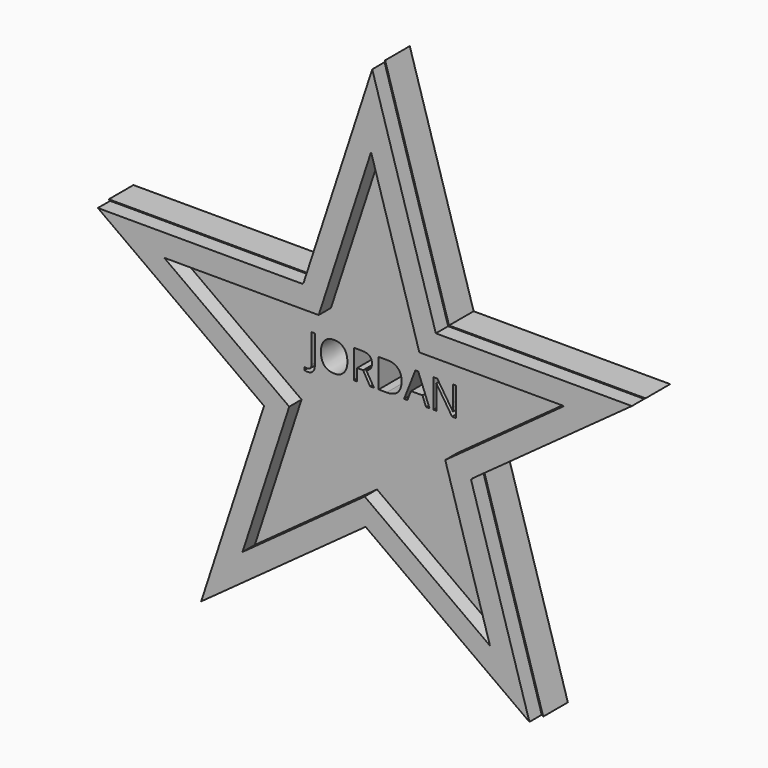
from build123d import *

# Parameters (mm, degrees)
F1_DEPTH = 6.35
F3_DEPTH = 3.175


with BuildPart() as f1:
    # F0 (on Front) → F1 (new body)
    with BuildSketch(Plane.XZ):
        Polygon((36.4045640823, 1.9488933967), (69.6907226001, 26.065217087), (29.1461811696, 26.1190709712), (15.9708538221, 69.9924798862), (1.6629783111, 26.15557594), (-41.0424164863, 26.2123000095), (-6.4774139305, 1.2147947246), (-19.4446871391, -38.5147311336), (14.4759376997, -13.9387270281), (48.5830571498, -38.6050899867), align=None)
        with BuildLine():
            add(Edge.make_bspline(
                [(1.0703261445, 8.6234759039), (0.6811166374, 8.1998862237), (-0.0492998709, 8.1998862237)],
                knots=[0, 0, 0, 1, 1, 1], degree=2))
            add(Edge.make_bspline(
                [(-0.0492998709, 8.1998862237), (-0.4294278228, 8.1998862237), (-0.6486825118, 8.3088648857)],
                knots=[0, 0, 0, 1, 1, 1], degree=2))
            Line((-0.6486825118, 8.3088648857), (-0.6486825118, 8.8965712414))
            add(Edge.make_bspline(
                [(-0.6486825118, 8.8965712414), (-0.3606674766, 8.81613461), (-0.0492998709, 8.81613461)],
                knots=[0, 0, 0, 1, 1, 1], degree=2))
            add(Edge.make_bspline(
                [(-0.0492998709, 8.81613461), (0.3528832864, 8.81613461), (0.5617590552, 9.0593905519)],
                knots=[0, 0, 0, 1, 1, 1], degree=2))
            add(Edge.make_bspline(
                [(0.5617590552, 9.0593905519), (0.7706348241, 9.3026464938), (0.7706348241, 9.7606163472)],
                knots=[0, 0, 0, 1, 1, 1], degree=2))
            Line((0.7706348241, 9.7606163472), (0.7706348241, 15.6882771403))
            Line((0.7706348241, 15.6882771403), (1.4595356516, 15.6882771403))
            Line((1.4595356516, 15.6882771403), (1.4595356516, 9.8177004082))
            add(Edge.make_bspline(
                [(1.4595356516, 9.8177004082), (1.4595356516, 9.0470655842), (1.0703261445, 8.6234759039)],
                knots=[0, 0, 0, 1, 1, 1], degree=2))
        make_face(mode=Mode.SUBTRACT)
        with BuildLine():
            add(Edge.make_bspline(
                [(7.4598488861, 14.9708342823), (8.1772917442, 14.1599811425), (8.1772917442, 12.7328796164)],
                knots=[0, 0, 0, 1, 1, 1], degree=2))
            add(Edge.make_bspline(
                [(8.1772917442, 12.7328796164), (8.1772917442, 11.3096701855), (7.4572541561, 10.4942762681)],
                knots=[0, 0, 0, 1, 1, 1], degree=2))
            add(Edge.make_bspline(
                [(7.4572541561, 10.4942762681), (6.7372165679, 9.6788823507), (5.4567172896, 9.6788823507)],
                knots=[0, 0, 0, 1, 1, 1], degree=2))
            add(Edge.make_bspline(
                [(5.4567172896, 9.6788823507), (4.1476759807, 9.6788823507), (3.4360712652, 10.4800052528)],
                knots=[0, 0, 0, 1, 1, 1], degree=2))
            add(Edge.make_bspline(
                [(3.4360712652, 10.4800052528), (2.7244665497, 11.2811281549), (2.7244665497, 12.7406638066)],
                knots=[0, 0, 0, 1, 1, 1], degree=2))
            add(Edge.make_bspline(
                [(2.7244665497, 12.7406638066), (2.7244665497, 14.188523173), (3.4380173127, 14.9851052975)],
                knots=[0, 0, 0, 1, 1, 1], degree=2))
            add(Edge.make_bspline(
                [(3.4380173127, 14.9851052975), (4.1515680757, 15.781687422), (5.4645014797, 15.781687422)],
                knots=[0, 0, 0, 1, 1, 1], degree=2))
            add(Edge.make_bspline(
                [(5.4645014797, 15.781687422), (6.742406028, 15.781687422), (7.4598488861, 14.9708342823)],
                knots=[0, 0, 0, 1, 1, 1], degree=2))
        make_face(mode=Mode.SUBTRACT)
        with BuildLine():
            Line((11.4245963984, 12.2256098922), (10.1869101659, 12.2256098922))
            Line((10.1869101659, 12.2256098922), (10.1869101659, 9.7606163472))
            Line((10.1869101659, 9.7606163472), (9.4980093383, 9.7606163472))
            Line((9.4980093383, 9.7606163472), (9.4980093383, 15.6882771403))
            Line((9.4980093383, 15.6882771403), (11.1236077129, 15.6882771403))
            add(Edge.make_bspline(
                [(11.1236077129, 15.6882771403), (12.2146916979, 15.6882771403), (12.7355837549, 15.2705256027)],
                knots=[0, 0, 0, 1, 1, 1], degree=2))
            add(Edge.make_bspline(
                [(12.7355837549, 15.2705256027), (13.2564758119, 14.8527740651), (13.2564758119, 14.0133788948)],
                knots=[0, 0, 0, 1, 1, 1], degree=2))
            add(Edge.make_bspline(
                [(13.2564758119, 14.0133788948), (13.2564758119, 12.8379661833), (12.0641973551, 12.4241067408)],
                knots=[0, 0, 0, 1, 1, 1], degree=2))
            Line((12.0641973551, 12.4241067408), (13.6742273495, 9.7606163472))
            Line((13.6742273495, 9.7606163472), (12.8594821146, 9.7606163472))
            Line((12.8594821146, 9.7606163472), (11.4245963984, 12.2256098922))
        make_face(mode=Mode.SUBTRACT)
        with BuildLine():
            add(Edge.make_bspline(
                [(18.5957815668, 14.9221830939), (19.3618756133, 14.1560890474), (19.3618756133, 12.7808821223)],
                knots=[0, 0, 0, 1, 1, 1], degree=2))
            add(Edge.make_bspline(
                [(19.3618756133, 12.7808821223), (19.3618756133, 11.3135622805), (18.5652934887, 10.5370893139)],
                knots=[0, 0, 0, 1, 1, 1], degree=2))
            add(Edge.make_bspline(
                [(18.5652934887, 10.5370893139), (17.7687113642, 9.7606163472), (16.2728494919, 9.7606163472)],
                knots=[0, 0, 0, 1, 1, 1], degree=2))
            Line((16.2728494919, 9.7606163472), (14.6303853719, 9.7606163472))
            Line((14.6303853719, 9.7606163472), (14.6303853719, 15.6882771403))
            Line((14.6303853719, 15.6882771403), (16.4466964051, 15.6882771403))
            add(Edge.make_bspline(
                [(16.4466964051, 15.6882771403), (17.8296875203, 15.6882771403), (18.5957815668, 14.9221830939)],
                knots=[0, 0, 0, 1, 1, 1], degree=2))
        make_face(mode=Mode.SUBTRACT)
        Polygon((25.1234736834, 9.7606163472), (24.4099229204, 9.7606163472), (23.6717222219, 11.6456877266), (21.2962468635, 11.6456877266), (20.5671277202, 9.7606163472), (19.8691453375, 9.7606163472), (22.2121865703, 15.7129270758), (22.7921087358, 15.7129270758), align=None, mode=Mode.SUBTRACT)
        with BuildLine():
            Line((30.5685146877, 15.6882771403), (30.5685146877, 9.7606163472))
            Line((30.5685146877, 9.7606163472), (29.7823114834, 9.7606163472))
            Line((29.7823114834, 9.7606163472), (26.5427910193, 14.7347138479))
            Line((26.5427910193, 14.7347138479), (26.5103568937, 14.7347138479))
            add(Edge.make_bspline(
                [(26.5103568937, 14.7347138479), (26.5752251449, 13.858992457), (26.5752251449, 13.1298733137)],
                knots=[0, 0, 0, 1, 1, 1], degree=2))
            Line((26.5752251449, 13.1298733137), (26.5752251449, 9.7606163472))
            Line((26.5752251449, 9.7606163472), (25.9382189182, 9.7606163472))
            Line((25.9382189182, 9.7606163472), (25.9382189182, 15.6882771403))
            Line((25.9382189182, 15.6882771403), (26.7166379324, 15.6882771403))
            Line((26.7166379324, 15.6882771403), (29.9483742064, 10.7336401149))
            Line((29.9483742064, 10.7336401149), (29.980808332, 10.7336401149))
            add(Edge.make_bspline(
                [(29.980808332, 10.7336401149), (29.9730241418, 10.8426187769), (29.9444821113, 11.4368119578)],
                knots=[0, 0, 0, 1, 1, 1], degree=2))
            add(Edge.make_bspline(
                [(29.9444821113, 11.4368119578), (29.9159400808, 12.0310051386), (29.9237242709, 12.2865860483)],
                knots=[0, 0, 0, 1, 1, 1], degree=2))
            Line((29.9237242709, 12.2865860483), (29.9237242709, 15.6882771403))
            Line((29.9237242709, 15.6882771403), (30.5685146877, 15.6882771403))
        make_face(mode=Mode.SUBTRACT)
    extrude(amount=F1_DEPTH)

    # F2 (on face) → F3 (join)
    with BuildSketch(Plane.XZ.offset(6.35)):
        Polygon((36.4045640823, 1.9488933967), (69.4127031084, 25.8637877737), (28.9641653483, 25.9175141396), (15.8445339726, 69.6054572911), (1.6629783111, 26.15557594), (1.5467987544, 26.1557302572), (1.4809624898, 25.9540191084), (-40.7628684516, 26.0101300989), (-6.4774139305, 1.2147947246), (-19.4446871391, -38.5147311336), (14.4759376997, -13.9387270281), (48.2732234246, -38.3810173811), (36.222548261, 1.7473365651), (36.421750894, 1.891661876), align=None)
        Polygon((55.4314800111, 21.3103554065), (30.9093811696, 3.5437250843), (40.1384522175, -27.1887794914), (14.2914917683, -8.4961863292), (-10.9143527112, -26.7582006747), (-1.2785905938, 2.7641402252), (-27.0746829363, 21.4199454322), (4.7966385236, 21.3776118802), (15.6072232815, 54.4994101005), (25.5620899488, 21.3500298636), align=None, mode=Mode.SUBTRACT)
    extrude(amount=F3_DEPTH)


solid = f1.part
